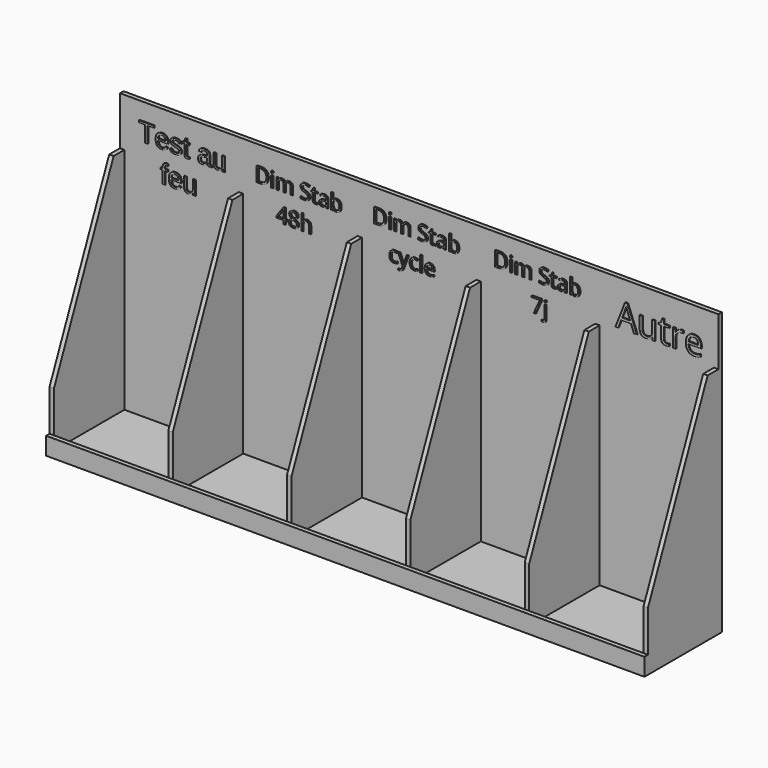
from build123d import *

# Parameters (mm, degrees)
F0_W            = 3400
F0_H            = 500
F1_DEPTH        = 25
F2_W            = 25
F2_H            = 500
F3_DEPTH        = 1300
F4_W            = 3400
F4_H            = 1600
F5_DEPTH        = 25
F7_DEPTH        = 3400
F8_W            = 3400
F8_H            = 100
F9_DEPTH        = 25
F10_TEXT_SIZE   = 149.805720706
F10_TEXT_SIZE_2 = 117.5908573108
F10_TEXT_SIZE_3 = 193.6928757339
F11_DEPTH       = 5


# Not quite as in the source:
# - Text() gives the source's letters only with a copy of the font that has no kerning and outlines rounded to 1/6400 em; it was checked with that copy


with BuildPart() as f1:
    # F0 (on Top) → F1 (new body)
    with BuildSketch(Plane.XY):
        with Locations((1700, 250)):
            Rectangle(F0_W, F0_H)
    extrude(amount=F1_DEPTH)

    # F2 (on face) → F3 (join)
    with BuildSketch(Plane.XY.offset(25)):
        with Locations((12.5, 250)):
            Rectangle(F2_W, F2_H)
        with Locations((687.5, 250)):
            Rectangle(F2_W, F2_H)
        with Locations((1362.5, 250)):
            Rectangle(F2_W, F2_H)
        with Locations((2037.5, 250)):
            Rectangle(F2_W, F2_H)
        with Locations((2712.5, 250)):
            Rectangle(F2_W, F2_H)
        with Locations((3387.5, 250)):
            Rectangle(F2_W, F2_H)
    extrude(amount=F3_DEPTH)

    # F4 (on face) → F5 (join)
    with BuildSketch(Plane(origin=(0, 500, 0), x_dir=(-1, 0, 0), z_dir=(0, 1, 0))):
        with Locations((-1700, 800)):
            Rectangle(F4_W, F4_H)
    extrude(amount=F5_DEPTH)

    # F6 (on face) → F7 (cut, through all)
    with BuildSketch(Plane(origin=(0, 0, 0), x_dir=(0, -1, 0), z_dir=(-1, 0, 0))):
        Polygon((0, 335.7991576195), (0, 1325), (-423.537582159, 1325), align=None)
    extrude(amount=-F7_DEPTH, mode=Mode.SUBTRACT)

    # F8 (on face) → F9 (join)
    with BuildSketch(Plane.XZ):
        with Locations((1700, 50)):
            Rectangle(F8_W, F8_H)
    extrude(amount=F9_DEPTH)


with BuildPart() as f11:
    # F10 (on face) → F11 (new body)
    with BuildSketch(Plane.XZ.offset(-500)):
        with Locations((108.4442047064, 1400.1498479855)):
            Text('Test au', F10_TEXT_SIZE, font='Arimo', text_align=(TextAlign.LEFT, TextAlign.BOTTOM))
        with Locations((233.2979100573, 1227.8732691737)):
            Text('feu', F10_TEXT_SIZE, font='Arimo', text_align=(TextAlign.LEFT, TextAlign.BOTTOM))
        with Locations((767.3194408417, 1409.2855457565)):
            Text('Dim Stab', F10_TEXT_SIZE_2, font='Open Sans', text_align=(TextAlign.LEFT, TextAlign.BOTTOM))
        with Locations((889.5404381591, 1249.3619798138)):
            Text('48h', F10_TEXT_SIZE_2, font='Open Sans', text_align=(TextAlign.LEFT, TextAlign.BOTTOM))
        with Locations((1436.0585212708, 1419.901132991)):
            Text('Dim Stab', F10_TEXT_SIZE_2, font='Open Sans', text_align=(TextAlign.LEFT, TextAlign.BOTTOM))
        with Locations((1527.7242692588, 1259.9775670483)):
            Text('cycle', F10_TEXT_SIZE_2, font='Open Sans', text_align=(TextAlign.LEFT, TextAlign.BOTTOM))
        with Locations((2123.6987113953, 1427.2555116913)):
            Text('Dim Stab', F10_TEXT_SIZE_2, font='Open Sans', text_align=(TextAlign.LEFT, TextAlign.BOTTOM))
        with Locations((2337.5854567008, 1267.3319457485)):
            Text('7j', F10_TEXT_SIZE_2, font='Open Sans', text_align=(TextAlign.LEFT, TextAlign.BOTTOM))
        with Locations((2818.6931610107, 1350.3986839073)):
            Text('Autre', F10_TEXT_SIZE_3, font='Open Sans', text_align=(TextAlign.LEFT, TextAlign.BOTTOM))
    extrude(amount=F11_DEPTH)


solid = Compound([f1.part, f11.part])
